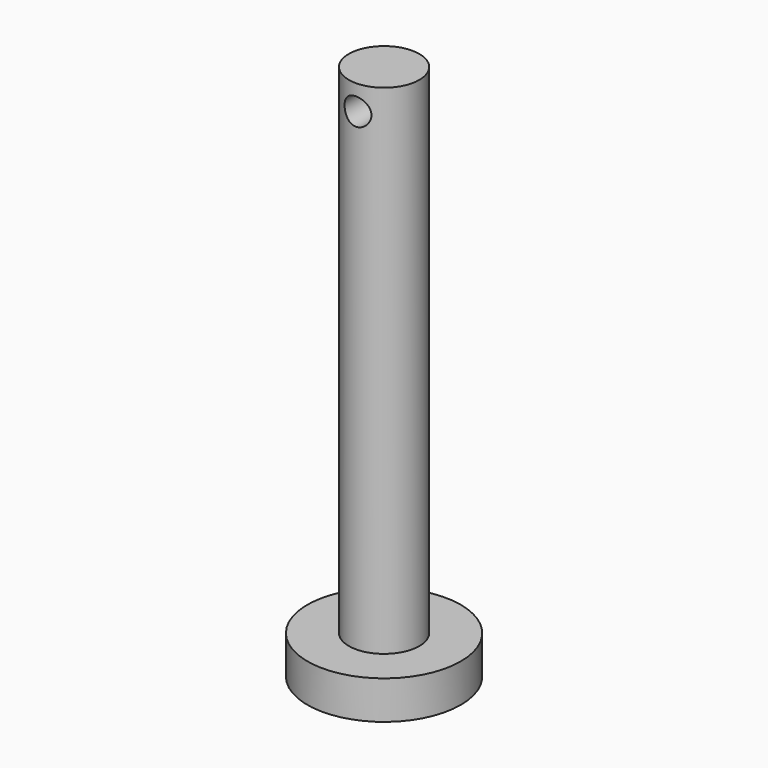
from build123d import *

# Parameters (mm, degrees)
F0_R     = 2.335
F1_DEPTH = 33.02
F2_R     = 5.08
F2_R_2   = 2.335
F3_DEPTH = 2.54
F4_R     = 0.889
F5_DEPTH = 12.7


with BuildPart() as f1:
    # F0 (on Top) → F1 (new body)
    with BuildSketch(Plane.XY):
        Circle(F0_R)
    extrude(amount=F1_DEPTH)

    # F2 (on face) → F3 (join)
    with BuildSketch(Plane(origin=(0, 0, 0), x_dir=(1, 0, 0), z_dir=(0, 0, -1))):
        Circle(F2_R)
        Circle(F2_R_2, mode=Mode.SUBTRACT)
        Circle(F2_R_2)
    extrude(amount=F3_DEPTH)

    # F4 (on Front) → F5 (cut, symmetric)
    with BuildSketch(Plane.XZ):
        with Locations((0, 31.369)):
            Circle(F4_R)
    extrude(amount=F5_DEPTH, both=True, mode=Mode.SUBTRACT)


solid = f1.part
